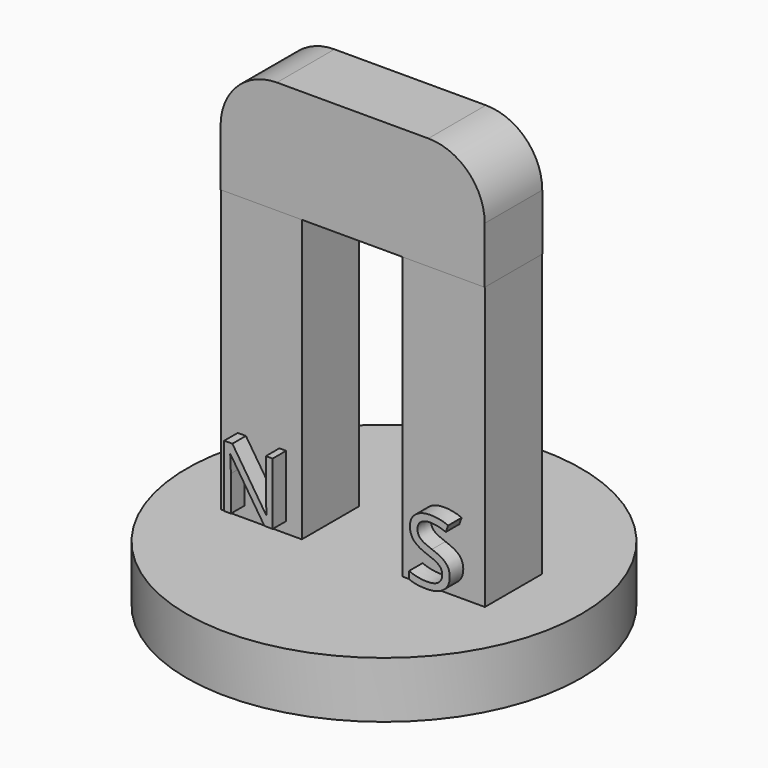
from build123d import *

# Parameters (mm, degrees)
F0_R           = 17.5
F1_DEPTH       = 5
F2_W           = 7.175214123
F2_H           = 6.3408871647
F2_W_2         = 7.3244892992
F3_DEPTH       = 25
F4_W           = 23.4410502017
F4_H           = 6.3829240971
F5_DEPTH       = 10
F6_R           = 5
F7_TEXT_SIZE   = 7.7022349514
F7_TEXT_SIZE_2 = 8.0298968694
F8_DEPTH       = 1.5


# Not quite as in the source:
# - Text() gives the source's letters only with a copy of the font that has no kerning and outlines rounded to 1/6400 em; it was checked with that copy


with BuildPart() as f1:
    # F0 (on Top) → F1 (new body)
    with BuildSketch(Plane.XY):
        Circle(F0_R)
    extrude(amount=F1_DEPTH)

    # F2 (on face) → F3 (join)
    with BuildSketch(Plane.XY.offset(5)):
        with Locations((-8.2166327629, -0.1603244455)):
            Rectangle(F2_W, F2_H)
        with Locations((7.9572868999, -0.1603244455)):
            Rectangle(F2_W_2, F2_H)
    extrude(amount=F3_DEPTH)

    # F4 (on face) → F5 (join)
    with BuildSketch(Plane.XY.offset(30)):
        with Locations((-0.0837147236, -0.1813429117)):
            Rectangle(F4_W, F4_H)
    extrude(amount=F5_DEPTH)

    # F6
    f6_edges = [f1.edges().sort_by_distance(p)[0] for p in [
        (11.63681, -0.181343, 40),
        (-11.80424, -0.181343, 40),
    ]]
    fillet(f6_edges, radius=F6_R)

    # F7 (on face) → F8 (join)
    with BuildSketch(Plane.XZ.offset(3.3307680278)):
        with Locations((-11.0683627427, 5.970756989)):
            Text('N', F7_TEXT_SIZE, font='Open Sans', text_align=(TextAlign.LEFT, TextAlign.BOTTOM))
        with Locations((5.6776511483, 5.8052428067)):
            Text('S', F7_TEXT_SIZE_2, font='Open Sans', text_align=(TextAlign.LEFT, TextAlign.BOTTOM))
    extrude(amount=F8_DEPTH)


solid = f1.part
